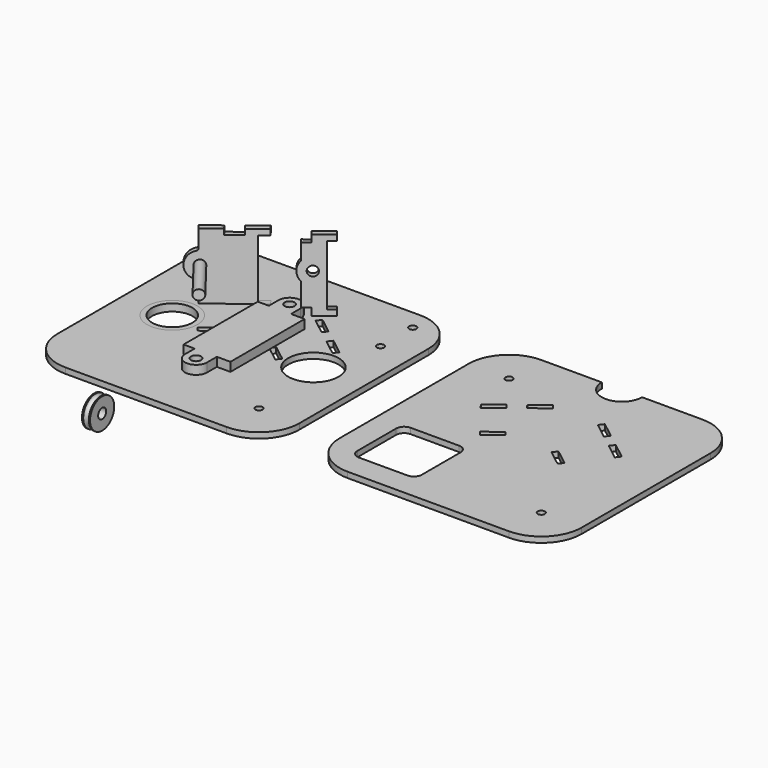
from build123d import *

# Parameters (mm, degrees)
F0_R      = 1.1294208385
F0_R_2    = 1.27
F0_R_3    = 7.9375
F0_R_4    = 1.1354051666
F0_R_5    = 1.143
F1_DEPTH  = 1.778
F2_R      = 1.524
F2_W      = 6.35
F2_H      = 1.778
F3_DEPTH  = 1.778
F7_R      = 1.5875
F8_DEPTH  = 26.9785760814
F14_R     = 7.9375
F14_R_2   = 6.35
F15_DEPTH = 2.286
F16_R     = 1.5875
F17_DEPTH = 2.794
F18_W     = 20.32
F18_H     = 20.32
F19_DEPTH = 0.762
F22_DEPTH = 2.286
F26_DEPTH = 55.2677051106
F30_R     = 8.8945160101
F30_R_2   = 8.6750306103
F30_W     = 11.43
F30_H     = 25.4
F30_R_3   = 1.3810752144
F30_R_4   = 2.4027367318
F30_R_5   = 2.4722571393
F30_R_6   = 2.9600908679
F31_DEPTH = 1.778
F32_R     = 6.35
F33_DEPTH = 4.319
F27_W     = 2.54
F27_H     = 7.4849529192
F27_H_2   = 5.954041196
F34_DEPTH = 1.778
F28_R     = 1.5705105082
F35_DEPTH = 15.875


# Not quite as in the source:
# - a feature names something its author has since deleted; it is built from what else it names


with BuildPart() as f1:
    # F0 (on Top) → F1 (new body)
    with BuildSketch(Plane.XY):
        with BuildLine():
            Line((27.9221547362, 61.3219190061), (-22.8778452638, 61.3219190061))
            ThreePointArc((-22.8778452638, 61.3219190061), (-31.8581013848, 57.6021751272), (-35.5778452638, 48.6219190061))
            Line((-35.5778452638, 48.6219190061), (-35.5778452638, 25.4619911658))
            Line((-35.5778452638, 25.4619911658), (-35.5778452638, 23.1759911658))
            Line((-35.5778452638, 23.1759911658), (-35.5778452638, -2.1780809939))
            ThreePointArc((-35.5778452638, -2.1780809939), (-31.8581013848, -11.158337115), (-22.8778452638, -14.8780809939))
            Line((-22.8778452638, -14.8780809939), (27.9221547362, -14.8780809939))
            ThreePointArc((27.9221547362, -14.8780809939), (36.9024108573, -11.158337115), (40.6221547362, -2.1780809939))
            Line((40.6221547362, -2.1780809939), (40.6221547362, 22.4352180958))
            Line((40.6221547362, 22.4352180958), (40.6221547362, 24.7212180958))
            Line((40.6221547362, 24.7212180958), (40.6221547362, 48.6219190061))
            ThreePointArc((40.6221547362, 48.6219190061), (36.9024108573, 57.6021751272), (27.9221547362, 61.3219190061))
        make_face()
        with Locations((27.9221547362, -2.1780809939)):
            Circle(F0_R, mode=Mode.SUBTRACT)
        with Locations((2.5221547362, 4.8069190061)):
            Circle(F0_R_2, mode=Mode.SUBTRACT)
        with Locations((-19.7028452638, 23.2219190061)):
            Circle(F0_R_3, mode=Mode.SUBTRACT)
        Polygon((-14.662863261, 37.4058066077), (-13.5741758307, 36.0000884001), (-18.5945980005, 32.1119190061), (-19.6832854309, 33.5176372137), align=None, mode=Mode.SUBTRACT)
        Polygon((-10.8182592125, 22.0710746664), (-5.7978370427, 25.9592440605), (-4.7091496123, 24.5535258529), (-9.7295717822, 20.6653564589), align=None, mode=Mode.SUBTRACT)
        Polygon((-4.537415925, 42.9987933094), (-9.5578380948, 39.1106239153), (-10.6465255252, 40.5163421229), (-5.6261033553, 44.4045115169), align=None, mode=Mode.SUBTRACT)
        with Locations((-22.8778452638, 48.6219190061)):
            Circle(F0_R_4, mode=Mode.SUBTRACT)
        Polygon((-3.1928452638, 35.9219190061), (2.5221547362, 35.9219190061), (3.3085793257, 35.9219190061), (8.2371547362, 35.9219190061), (8.2371547362, 10.5219190061), (2.5221547362, 10.5219190061), (-3.1928452638, 10.5219190061), align=None, mode=Mode.SUBTRACT)
        Polygon((14.7738812547, 20.6653564589), (9.7534590848, 24.5535258529), (10.8421465151, 25.9592440605), (15.862568685, 22.0710746664), align=None, mode=Mode.SUBTRACT)
        with Locations((2.5221547362, 41.6369190061)):
            Circle(F0_R_2, mode=Mode.SUBTRACT)
        Polygon((15.6908349976, 40.5163421229), (14.6021475673, 39.1106239153), (9.5817253975, 42.9987933094), (10.6704128278, 44.4045115169), align=None, mode=Mode.SUBTRACT)
        with Locations((24.7471547362, 23.2219190061)):
            Circle(F0_R_3, mode=Mode.SUBTRACT)
        Polygon((23.638907473, 32.1119190061), (18.6184853032, 36.0000884001), (19.7071727335, 37.4058066077), (24.7275949034, 33.5176372137), align=None, mode=Mode.SUBTRACT)
        with Locations((30.5796239127, 42.3334268199)):
            Circle(F0_R_5, mode=Mode.SUBTRACT)
        with Locations((30.5796239127, 55.0334268199)):
            Circle(F0_R_5, mode=Mode.SUBTRACT)
    extrude(amount=F1_DEPTH)


with BuildPart() as f3:
    # F2 (on face) → F3 (new body)
    with BuildSketch(Plane(origin=(-23.6057262531, 30.4798220979, 0), x_dir=(0.7906176645, 0.6123101408, 0), z_dir=(0.6123101408, -0.7906176645, 0))):
        with BuildLine():
            Line((4.9612360034, 7.9612624765), (4.9612360034, 2.2859991465))
            Line((4.9612360034, 2.2859991465), (4.9612360034, 1.778))
            Line((4.9612360034, 1.778), (11.3112360034, 1.778))
            Line((11.3112360034, 1.778), (16.3912360034, 1.778))
            Line((16.3912360034, 1.778), (16.3912360034, 0))
            Line((16.3912360034, 0), (22.7412360034, 0))
            Line((22.7412360034, 0), (22.7412360034, 1.778))
            Line((22.7412360034, 1.778), (19.5662360034, 1.778))
            Line((19.5662360034, 1.778), (19.5662360034, 20.828))
            Line((19.5662360034, 20.828), (22.7412360034, 20.828))
            Line((22.7412360034, 20.828), (22.7412360034, 22.606))
            Line((22.7412360034, 22.606), (16.3912360034, 22.606))
            Line((16.3912360034, 22.606), (16.3912360034, 20.828))
            Line((16.3912360034, 20.828), (11.3112360034, 20.828))
            Line((11.3112360034, 20.828), (11.3112360034, 22.606))
            Line((11.3112360034, 22.606), (4.9612360034, 22.606))
            Line((4.9612360034, 22.606), (4.9612360034, 16.9307358166))
            ThreePointArc((4.9612360034, 16.9307358166), (4.8458191864, 16.6083347552), (4.5520137812, 16.4324317422))
            ThreePointArc((4.5520137812, 16.4324317422), (1.2782360034, 12.4459991465), (4.5520137812, 8.4595665509))
            ThreePointArc((4.5520137812, 8.4595665509), (4.8458191864, 8.2836635379), (4.9612360034, 7.9612624765))
        make_face()
        with Locations((5.3422360034, 12.4459991465)):
            Circle(F2_R, mode=Mode.SUBTRACT)
        with Locations((8.1362360034, 0.889)):
            Rectangle(F2_W, F2_H)
    extrude(amount=F3_DEPTH)


with BuildPart() as f4_1:
    # F4: copy of F3
    add(f3.part.moved(Location((0, -13.97, 0))))


with BuildPart() as f6:
    # F5 (on Top) → F6 (revolve)
    with BuildSketch(Plane.XY):
        with BuildLine():
            Line((-11.1402691823, -31.1776632922), (-11.1402691823, -35.9401632922))
            Line((-11.1402691823, -35.9401632922), (-8.6002691823, -35.9401632922))
            Line((-8.6002691823, -35.9401632922), (-8.6002691823, -31.1776632922))
            Line((-8.6002691823, -31.1776632922), (-8.9812691823, -31.1776632922))
            ThreePointArc((-8.9812691823, -31.1776632922), (-9.8702691823, -32.0666632922), (-10.7592691823, -31.1776632922))
            Line((-10.7592691823, -31.1776632922), (-11.1402691823, -31.1776632922))
        make_face()
    revolve(axis=Axis((-9.8702691823, -35.9401632922, 0), (1, 0, 0)))

    # F7 (on face) → F8 (cut, through all)
    with BuildSketch(Plane.YZ.offset(-8.6002691823)):
        with Locations((-35.9401632922, 0)):
            Circle(F7_R)
    extrude(amount=-F8_DEPTH, mode=Mode.SUBTRACT)


with BuildPart() as f6_1:
    # F9: moved
    add(f6.part.moved(Location((8.636, 6.8834, -0.3175))))


with BuildPart() as f10_1:
    # F10: copy of F6
    add(f6_1.part.moved(Location((33.528, 0, 0))))


with BuildPart() as f6_2:
    # F13: moved
    add(f6_1.part.moved(Location((0, 0, 2.54))))


with BuildPart() as f15:
    # F14 (on face) → F15 (new body)
    with BuildSketch(Plane.XY.offset(1.778)):
        with Locations((-19.7028452638, 23.2219190061)):
            Circle(F14_R)
        with Locations((-19.7028452638, 23.2219190061)):
            Circle(F14_R_2, mode=Mode.SUBTRACT)
    extrude(amount=-F15_DEPTH)


with BuildPart() as f17:
    # F16 (on face) → F17 (new body)
    with BuildSketch(Plane.XY.offset(1.778)):
        with BuildLine():
            Line((-0.9703452638, 37.8269190061), (-4.4628452638, 37.8269190061))
            Line((-4.4628452638, 37.8269190061), (-4.4628452638, 8.6169190061))
            Line((-4.4628452638, 8.6169190061), (-0.9703452638, 8.6169190061))
            Line((-0.9703452638, 8.6169190061), (-0.9703452638, 4.8069190061))
            ThreePointArc((-0.9703452638, 4.8069190061), (2.5221547362, 1.3144190061), (6.0146547362, 4.8069190061))
            Line((6.0146547362, 4.8069190061), (6.0146547362, 8.6169190061))
            Line((6.0146547362, 8.6169190061), (10.2935793257, 8.6169190061))
            Line((10.2935793257, 8.6169190061), (10.2935793257, 37.8269190061))
            Line((10.2935793257, 37.8269190061), (6.0146547362, 37.8269190061))
            Line((6.0146547362, 37.8269190061), (6.0146547362, 41.6369190061))
            ThreePointArc((6.0146547362, 41.6369190061), (2.5221547362, 45.1294190061), (-0.9703452638, 41.6369190061))
            Line((-0.9703452638, 41.6369190061), (-0.9703452638, 37.8269190061))
        make_face()
        with Locations((2.5221547362, 4.8069190061)):
            Circle(F16_R, mode=Mode.SUBTRACT)
        with Locations((2.5221547362, 41.6369190061)):
            Circle(F16_R, mode=Mode.SUBTRACT)
    extrude(amount=F17_DEPTH)


with BuildPart() as f19:
    # F18 (on Top) → F19 (new body)
    with BuildSketch(Plane.XY):
        with Locations((-51.0207973421, 12.4038157185)):
            Rectangle(F18_W, F18_H)
    extrude(amount=F19_DEPTH)


with BuildPart() as f22:
    # F22 (new): a face of the model
    f22_faces = [f1.part.faces().sort_by_distance(p)[0] for p in [
        (-17.1730743459, 35.4617219107, 0.889),
    ]]
    extrude(f22_faces, amount=F22_DEPTH)


with BuildPart() as f24_1:
    # F24: copy of F3
    add(f3.part.moved(Location((35.56, 0, 9.906))))

    # F25 (on face) → F26 (cut, through all)
    with BuildSketch(Plane(origin=(-9.184751748, 11.8593936188, 0), x_dir=(0.7906176645, 0.6123101408, 0), z_dir=(0.6123101408, -0.7906176645, 0))):
        Polygon((50.8556001545, 32.512), (39.4256001545, 32.512), (39.4256001545, 30.734), (36.8856001545, 30.734), (36.8856001545, 11.684), (39.4256001545, 11.684), (39.4256001545, 9.906), (50.8556001545, 9.906), align=None)
    extrude(amount=-F26_DEPTH, mode=Mode.SUBTRACT)

    # F27 (on face) → F34 (join)
    with BuildSketch(Plane(origin=(-9.184751748, 11.8593936188, 0), x_dir=(0.7906176645, 0.6123101408, 0), z_dir=(0.6123101408, -0.7906176645, 0))):
        with Locations((31.8056001545, 15.9344764596)):
            Rectangle(F27_W, F27_H)
        with Locations((31.8056001545, 27.248979402)):
            Rectangle(F27_W, F27_H_2)
    extrude(amount=-F34_DEPTH)


with BuildPart() as f29_1:
    # F29: copy of F1
    add(f1.part.moved(Location((88.9, 0, 0))))

    # F30 (on face) → F31 (join)
    with BuildSketch(Plane.XY.offset(1.778)):
        with Locations((69.1971547362, 23.2219190061)):
            Circle(F30_R)
        with Locations((113.6471547362, 23.2219190061)):
            Circle(F30_R_2)
        with Locations((91.4221547362, 23.2219190061)):
            Rectangle(F30_W, F30_H)
        with Locations((91.4221547362, 41.6369190061)):
            Circle(F30_R_3)
        with Locations((119.4796239127, 42.3334268199)):
            Circle(F30_R_4)
        with Locations((119.4796239127, 55.0334268199)):
            Circle(F30_R_5)
        with Locations((91.4221547362, 4.8069190061)):
            Circle(F30_R_6)
    extrude(amount=-F31_DEPTH)

    # F32 (on face) → F33 (cut, through all)
    with BuildSketch(Plane.XY.offset(1.778)):
        with BuildLine():
            Line((78.7221547362, 13.0619190061), (63.4821547362, 13.0619190061))
            ThreePointArc((63.4821547362, 13.0619190061), (61.686103512, 12.3179702303), (60.9421547362, 10.5219190061))
            Line((60.9421547362, 10.5219190061), (60.9421547362, -4.7180809939))
            ThreePointArc((60.9421547362, -4.7180809939), (61.686103512, -6.5141322181), (63.4821547362, -7.2580809939))
            Line((63.4821547362, -7.2580809939), (78.7221547362, -7.2580809939))
            ThreePointArc((78.7221547362, -7.2580809939), (80.5182059605, -6.5141322181), (81.2621547362, -4.7180809939))
            Line((81.2621547362, -4.7180809939), (81.2621547362, 10.5219190061))
            ThreePointArc((81.2621547362, 10.5219190061), (80.5182059605, 12.3179702303), (78.7221547362, 13.0619190061))
        make_face()
        with Locations((91.4221547362, 61.3219190061)):
            Circle(F32_R)
    extrude(amount=-F33_DEPTH, mode=Mode.SUBTRACT)


with BuildPart() as f35:
    # F28 (on face) → F35 (new body)
    with BuildSketch(Plane(origin=(-22.5170388228, 29.0741038904, 0), x_dir=(0.7906176645, 0.6123101408, 0), z_dir=(0.6123101408, -0.7906176645, 0))):
        with Locations((5.3422360034, 12.4459991465)):
            Circle(F28_R)
    extrude(amount=F35_DEPTH)


solid = Compound([f1.part, f3.part, f6_2.part, f15.part, f17.part, f24_1.part, f29_1.part, f35.part])
